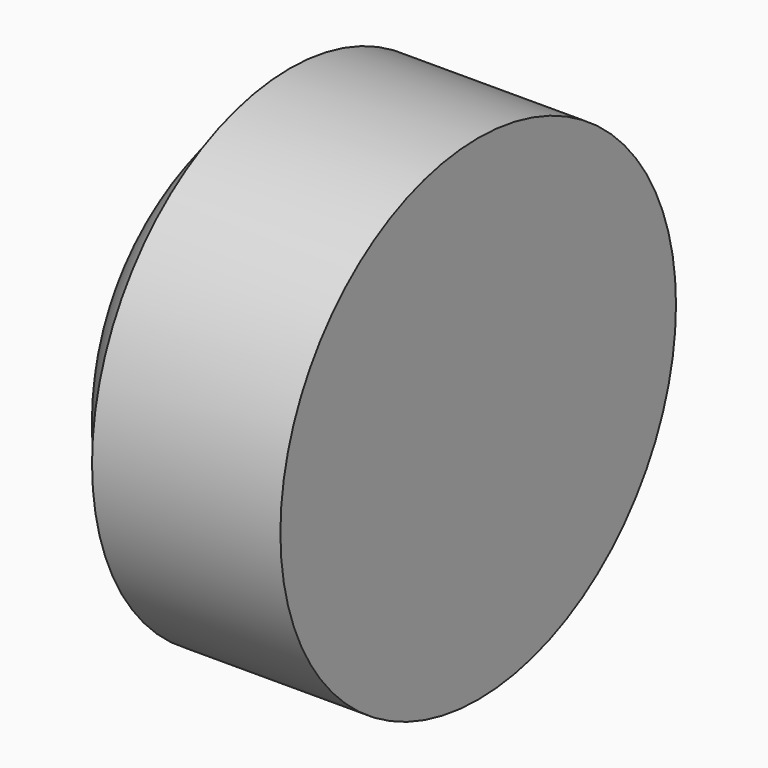
from build123d import *

# Parameters (mm, degrees)
F0_W   = 4
F0_H   = 5
F0_W_2 = 2
F0_H_2 = 0.25


# Not quite as in the source:
# - a fillet or chamfer that OpenCascade refuses, or shapes differently, is made with other operations: its cross-section is extruded or revolved along the edge and cut away or added


with BuildPart() as f1:
    # F0 (on Front) → F1 (revolve)
    with BuildSketch(Plane.XZ):
        with Locations((-2, 2.5)):
            Rectangle(F0_W, F0_H)
        with Locations((-5, 2.5)):
            Rectangle(F0_W_2, F0_H)
        with Locations((-2, 5.125)):
            Rectangle(F0_W, F0_H_2)
    revolve(axis=Axis((-3, 0, 0), (-1, 0, 0)))

    # F2: fillet of radius 5 on 1 edges, made by hand

    # F2_s1 → F2_t2 (revolve, cut)
    with BuildSketch(Plane.XZ):
        with BuildLine():
            ThreePointArc((-4, 5), (-5.472135955, 3.2360679775), (-6, 1))
            Line((-6, 1), (-6, 5))
            Line((-6, 5), (-4, 5))
        make_face()
    revolve(axis=Axis((-6, 0, 0), (-1, 0, 0)), mode=Mode.SUBTRACT)


solid = f1.part
